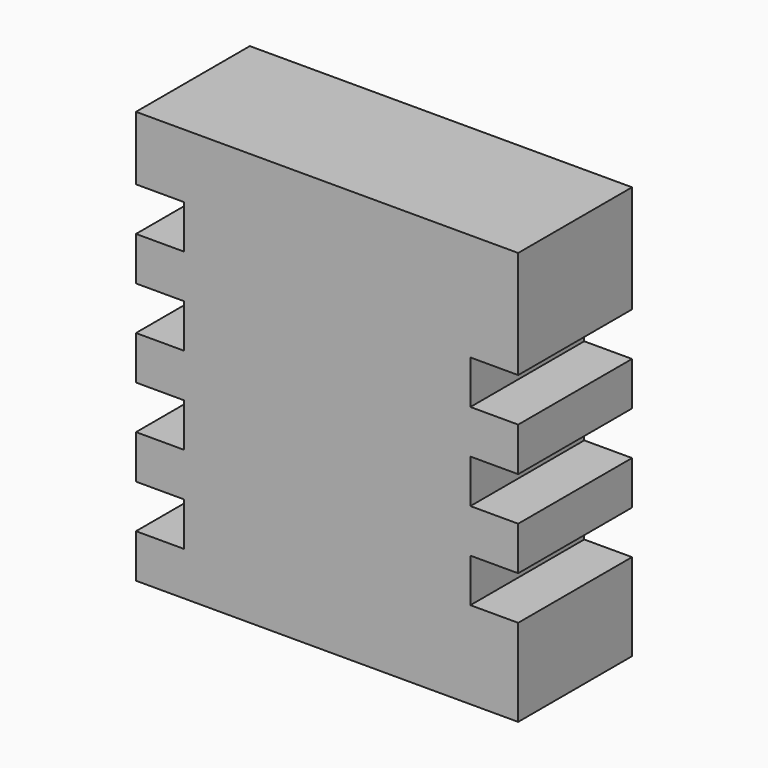
from build123d import *

# Parameters (mm, degrees)
F0_W     = 68.79
F0_H     = 25.61
F1_DEPTH = 25.61
F2_DEPTH = 100
F3_W     = 8.59875
F3_H     = 7.850625
F4_DEPTH = 50
F5_DEPTH = 51.308


with BuildPart() as f1:
    # F0 (on Top) → F1 (new body)
    with BuildSketch(Plane.XY):
        Rectangle(F0_W, F0_H)
    extrude(amount=F1_DEPTH)

    # F2 (add): a face of the model
    f2_faces = [f1.faces().sort_by_distance(p)[0] for p in [
        (0, 0, 0),
    ]]
    extrude(f2_faces, amount=F2_DEPTH)

    # F3 (on face) → F4 (cut)
    with BuildSketch(Plane.XZ.offset(12.805)):
        with Locations((-30.095625, -41.1203125)):
            Rectangle(F3_W, F3_H)
        with Locations((30.095625, -48.9709375)):
            Rectangle(F3_W, F3_H)
        with Locations((-30.095625, -56.8215625)):
            Rectangle(F3_W, F3_H)
        with Locations((30.095625, -64.6721875)):
            Rectangle(F3_W, F3_H)
        with Locations((-30.095625, -72.5228125)):
            Rectangle(F3_W, F3_H)
        with Locations((30.095625, -80.3734375)):
            Rectangle(F3_W, F3_H)
        with Locations((-30.095625, -88.2240625)):
            Rectangle(F3_W, F3_H)
    extrude(amount=-F4_DEPTH, mode=Mode.SUBTRACT)

    # F5 (cut): a face of the model
    f5_faces = [f1.faces().sort_by_distance(p)[0] for p in [
        (0, 0, 25.61),
    ]]
    extrude(f5_faces, amount=-F5_DEPTH, mode=Mode.SUBTRACT)


solid = f1.part
